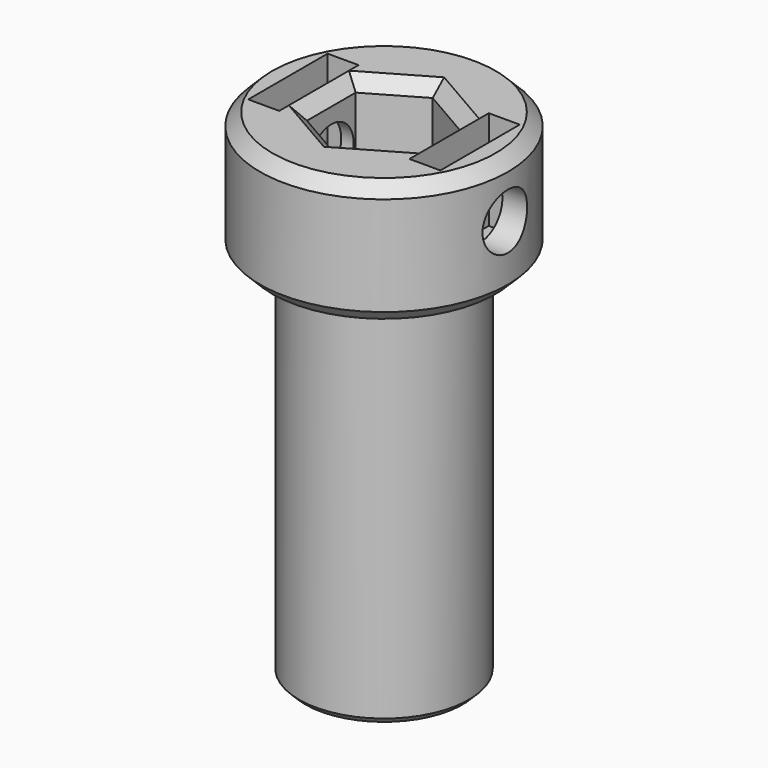
from build123d import *

# Parameters (mm, degrees)
F3_DEPTH = 40.001
F2_W     = 2.5
F2_H     = 8
F4_DEPTH = 8
F5_R     = 2.25
F6_DEPTH = 25
F7_SIZE  = 0.99999
F8_SIZE  = 0.5


# Not quite as in the source:
# - a fillet or chamfer is up to 0.001 mm smaller than in the source, because OpenCascade refuses the exact size


with BuildPart() as f1:
    # F0 (on Front) → F1 (revolve)
    with BuildSketch(Plane.XZ):
        Polygon((-6.85, 0), (0, 0), (0, 40), (-10, 40), (-10, 30), (-6.85, 30), align=None)
    revolve(axis=Axis((0, 0, 20), (0, 0, -1)))

    # F2 (on face) → F3 (cut, through all)
    with BuildSketch(Plane.XY.offset(40)):
        Polygon((4.25, -2.4537386441), (4.25, 2.4537386441), (0, 4.9074772881), (-4.25, 2.4537386441), (-4.25, -2.4537386441), (0, -4.9074772881), align=None)
    extrude(amount=-F3_DEPTH, mode=Mode.SUBTRACT)

    # F2 (on face) → F4 (cut)
    with BuildSketch(Plane.XY.offset(40)):
        with Locations((-6.5, 0)):
            Rectangle(F2_W, F2_H)
        with Locations((6.5, 0)):
            Rectangle(F2_W, F2_H)
    extrude(amount=-F4_DEPTH, mode=Mode.SUBTRACT)

    # F5 (on face) → F6 (cut, symmetric)
    with BuildSketch(Plane(origin=(-5.25, 0, 0), x_dir=(0, -1, 0), z_dir=(-1, 0, 0))):
        with Locations((0, 35.5)):
            Circle(F5_R)
    extrude(amount=F6_DEPTH, both=True, mode=Mode.SUBTRACT)

    # F7 (size 1 in the source; OpenCascade refuses exactly that, so slightly less here)
    f7_edges = [f1.edges().sort_by_distance(p)[0] for p in [
        (10, 0, 40),
        (10, 0, 30),
        (-2.125, 3.680608, 40),
        (2.125, 3.680608, 40),
        (4.25, 0, 40),
        (2.125, -3.680608, 40),
        (-2.125, -3.680608, 40),
        (-4.25, 0, 40),
    ]]
    chamfer(f7_edges, length=F7_SIZE)

    # F8
    f8_edges = [f1.edges().sort_by_distance(p)[0] for p in [
        (6.85, 0, 0),
        (4.25, 0, 0),
        (2.125, -3.680608, 0),
        (-2.125, -3.680608, 0),
        (-4.25, 0, 0),
        (-2.125, 3.680608, 0),
        (2.125, 3.680608, 0),
    ]]
    chamfer(f8_edges, length=F8_SIZE)


solid = f1.part
